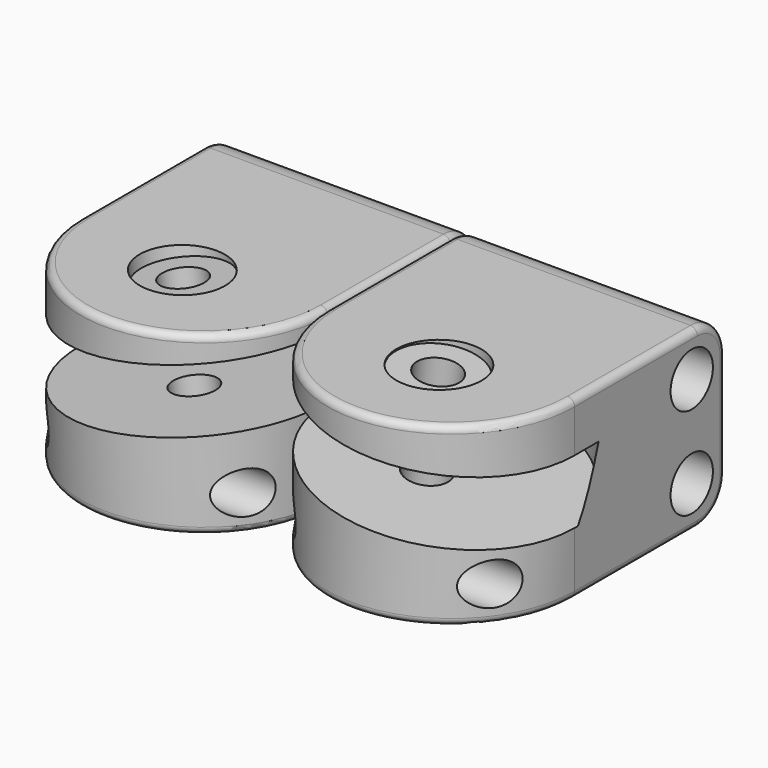
from build123d import *

# Parameters (mm, degrees)
F0_R          = 3
F0_R_2        = 3.75
F1_DEPTH      = 35
F2_DEPTH      = 25
F5_DEPTH      = 25
F5_DEPTH_BACK = 25
F6_DEPTH      = 5
F8_START      = 7
F7_R          = 6
F7_R_2        = 3
F8_DEPTH      = 9
F9_R          = 1
F10_S5_R      = 3.75
F10_T6_DEPTH  = 9
F10_S11_R     = 3.75
F10_T12_DEPTH = 9
F11_DEPTH     = 29.0800808224
F12_DEPTH     = 3
F13_START     = 26
F13_DEPTH     = 14


# Not quite as in the source:
# - a fillet or chamfer that OpenCascade refuses, or shapes differently, is made with other operations: its cross-section is extruded or revolved along the edge and cut away or added


with BuildPart() as f1:
    # F0 (on Right) → F1 (new body)
    with BuildSketch(Plane.YZ):
        with BuildLine():
            Line((17.766822055, 10.7994352999), (-22.233177945, 10.7994352999))
            Line((-22.233177945, 10.7994352999), (-22.233177945, -14.2005647001))
            Line((-22.233177945, -14.2005647001), (17.766822055, -14.2005647001))
            ThreePointArc((17.766822055, -14.2005647001), (21.3023559609, -12.7360986061), (22.766822055, -9.2005647001))
            Line((22.766822055, -9.2005647001), (22.766822055, 5.7994352999))
            ThreePointArc((22.766822055, 5.7994352999), (21.3023559609, 9.3349692058), (17.766822055, 10.7994352999))
        make_face()
        with Locations((-14.233177945, -9.2005647001)):
            Circle(F0_R, mode=Mode.SUBTRACT)
        with Locations((16.766822055, -8.2005647001)):
            Circle(F0_R_2, mode=Mode.SUBTRACT)
        with Locations((16.766822055, 4.7994352999)):
            Circle(F0_R_2, mode=Mode.SUBTRACT)
    extrude(amount=F1_DEPTH)

    # F0 (on Right) → F2 (join)
    with BuildSketch(Plane.YZ):
        with Locations((16.766822055, 4.7994352999)):
            Circle(F0_R_2)
        with Locations((16.766822055, 4.7994352999)):
            Circle(F0_R, mode=Mode.SUBTRACT)
        with Locations((16.766822055, -8.2005647001)):
            Circle(F0_R_2)
        with Locations((16.766822055, -8.2005647001)):
            Circle(F0_R, mode=Mode.SUBTRACT)
    extrude(amount=F2_DEPTH)

    # F3 (on Top) → F5 (cut, two sides)
    with BuildSketch(Plane.XY) as f5_sk:
        with BuildLine():
            Line((35, -26.8306802252), (35, -3.9818156511))
            ThreePointArc((35, -3.9818156511), (17.5, -21.4818156511), (0, -3.9818156511))
            Line((0, -3.9818156511), (0, -26.8306802252))
            Line((0, -26.8306802252), (35, -26.8306802252))
        make_face()
    extrude(amount=-F5_DEPTH, mode=Mode.SUBTRACT)
    extrude(f5_sk.sketch, amount=F5_DEPTH_BACK, mode=Mode.SUBTRACT)

    # F0 (on Right) → F6 (join)
    with BuildSketch(Plane.YZ):
        with Locations((16.766822055, 4.7994352999)):
            Circle(F0_R)
        with Locations((16.766822055, -8.2005647001)):
            Circle(F0_R)
    extrude(amount=F6_DEPTH)

    # F7 (on face) → F8 (cut)
    with BuildSketch(Plane(origin=(1.8261347197, 0, 14.8726737817), x_dir=(0.9925461516, 0, -0.1218693434), z_dir=(-0.1218693434, 0, -0.9925461516)).offset(F8_START)):
        with BuildLine():
            ThreePointArc((0, -2.0048082738), (21.3737990176, -11.4239200012), (35.730613496, 7))
            ThreePointArc((35.730613496, 7), (12.0874279744, 25.4239200012), (0, -2.0048082738))
        make_face()
        with Locations((16.730613496, 7)):
            Circle(F7_R, mode=Mode.SUBTRACT)
        with Locations((16.730613496, 7)):
            Circle(F7_R)
        with Locations((16.730613496, 7)):
            Circle(F7_R_2, mode=Mode.SUBTRACT)
        with Locations((16.730613496, 7)):
            Circle(F7_R_2)
    extrude(amount=F8_DEPTH, mode=Mode.SUBTRACT)

    # F9
    f9_edges = [f1.edges().sort_by_distance(p)[0] for p in [
        (0, 6.892503, -14.200565),
        (35, 6.892503, -14.200565),
        (0, 21.302356, -12.736099),
        (35, 21.302356, -12.736099),
        (35, 22.766822, -1.700565),
        (35, 21.302356, 9.334969),
        (35, 6.892503, 10.799435),
        (0, 6.892503, 10.799435),
        (0, 21.302356, 9.334969),
        (0, 22.766822, -1.700565),
        (17.5, -21.481816, 10.799435),
        (17.5, -21.481816, -14.200565),
    ]]
    fillet(f9_edges, radius=F9_R)

    # F10: chamfer of 2 on 2 edges, made by hand


with BuildPart() as f10_tool2:
    # F10_s3 → F10_t4 (revolve)
    with BuildSketch(Plane.XY.offset(4.7994352999)):
        Polygon((25, 21.766822055), (23, 19.766822055), (25, 19.766822055), align=None)
    revolve(axis=Axis((25, 16.766822055, 4.7994352999), (1, 0, 0)))

    # F10_s5 → F10_t6 (intersect, symmetric)
    with BuildSketch(Plane.YZ.offset(24)):
        with Locations((16.766822055, 4.7994352999)):
            Circle(F10_S5_R)
    extrude(amount=F10_T6_DEPTH, both=True, mode=Mode.INTERSECT)


with BuildPart() as f1_1:
    add(f1.part)

    # F10_t1: cut F10_tool2
    add(f10_tool2.part, mode=Mode.SUBTRACT)


with BuildPart() as f10_tool8:
    # F10_s9 → F10_t10 (revolve)
    with BuildSketch(Plane.XY.offset(-8.2005647001)):
        Polygon((25, 21.766822055), (23, 19.766822055), (25, 19.766822055), align=None)
    revolve(axis=Axis((25, 16.766822055, -8.2005647001), (1, 0, 0)))

    # F10_s11 → F10_t12 (intersect, symmetric)
    with BuildSketch(Plane.YZ.offset(24)):
        with Locations((16.766822055, -8.2005647001)):
            Circle(F10_S11_R)
    extrude(amount=F10_T12_DEPTH, both=True, mode=Mode.INTERSECT)


with BuildPart() as f1_2:
    add(f1_1.part)

    # F10_t7: cut F10_tool8
    add(f10_tool8.part, mode=Mode.SUBTRACT)

    # F7 (on face) → F11 (cut, through all)
    with BuildSketch(Plane(origin=(1.8261347197, 0, 14.8726737817), x_dir=(0.9925461516, 0, -0.1218693434), z_dir=(-0.1218693434, 0, -0.9925461516))):
        with Locations((16.730613496, 7)):
            Circle(F7_R_2)
    extrude(amount=F11_DEPTH, mode=Mode.SUBTRACT)

    # F7 (on face) → F12 (cut)
    with BuildSketch(Plane(origin=(1.8261347197, 0, 14.8726737817), x_dir=(0.9925461516, 0, -0.1218693434), z_dir=(-0.1218693434, 0, -0.9925461516))):
        with Locations((16.730613496, 7)):
            Circle(F7_R)
        with Locations((16.730613496, 7)):
            Circle(F7_R_2, mode=Mode.SUBTRACT)
    extrude(amount=F12_DEPTH, mode=Mode.SUBTRACT)

    # F7 (on face) → F13 (cut)
    with BuildSketch(Plane(origin=(1.8261347197, 0, 14.8726737817), x_dir=(0.9925461516, 0, -0.1218693434), z_dir=(-0.1218693434, 0, -0.9925461516)).offset(F13_START)):
        with Locations((16.730613496, 7)):
            Circle(F7_R)
        with Locations((16.730613496, 7)):
            Circle(F7_R_2, mode=Mode.SUBTRACT)
    extrude(amount=F13_DEPTH, mode=Mode.SUBTRACT)


with BuildPart() as f14_1:
    # F14: instance of F1
    add(f1_2.part.mirror(Plane.YZ))


solid = Compound([f1_2.part, f14_1.part])
